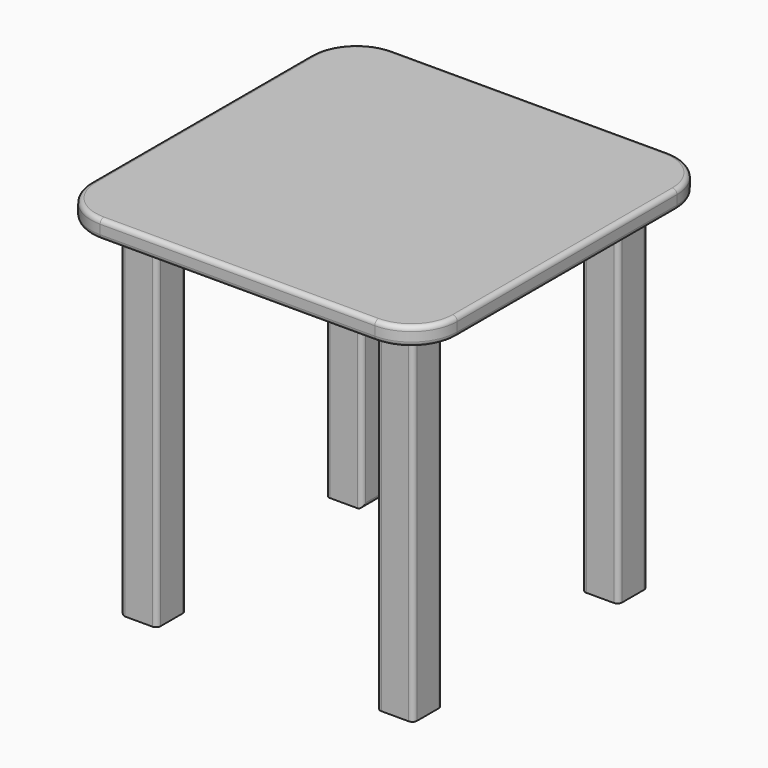
from build123d import *

# Parameters (mm, degrees)
F1_DEPTH = 20
F2_R     = 5
F3_W     = 40
F3_H     = 40
F4_DEPTH = 380
F5_F1_R  = 5
F5_F2_R  = 5
F6_R     = 5


with BuildPart() as f1:
    # F0 (on Top) → F1 (new body)
    with BuildSketch(Plane.XY):
        with BuildLine():
            Line((105.9260419756, 203.463898824), (-194.0739580244, 203.463898824))
            ThreePointArc((-194.0739580244, 203.463898824), (-229.4292970837, 188.8192378834), (-244.0739580244, 153.463898824))
            Line((-244.0739580244, 153.463898824), (-244.0739580244, -146.536101176))
            ThreePointArc((-244.0739580244, -146.536101176), (-229.4292970837, -181.8914402353), (-194.0739580244, -196.536101176))
            Line((-194.0739580244, -196.536101176), (105.9260419756, -196.536101176))
            ThreePointArc((105.9260419756, -196.536101176), (141.2813810349, -181.8914402353), (155.9260419756, -146.536101176))
            Line((155.9260419756, -146.536101176), (155.9260419756, 153.463898824))
            ThreePointArc((155.9260419756, 153.463898824), (141.2813810349, 188.8192378834), (105.9260419756, 203.463898824))
        make_face()
    extrude(amount=F1_DEPTH)

    # F2
    f2_edges = [f1.edges().sort_by_distance(p)[0] for p in [
        (-44.073958, 203.463899, 0),
        (-229.429297, 188.819238, 0),
        (-244.073958, 3.463899, 0),
        (-229.429297, -181.89144, 0),
        (-44.073958, -196.536101, 0),
        (141.281381, -181.89144, 0),
        (155.926042, 3.463899, 0),
        (141.281381, 188.819238, 0),
    ]]
    fillet(f2_edges, radius=F2_R)

    # F3 (on face) → F4 (join)
    with BuildSketch(Plane(origin=(0, 0, 0), x_dir=(1, 0, 0), z_dir=(0, 0, -1))):
        with Locations((95.9260419756, 136.536101176)):
            Rectangle(F3_W, F3_H)
        with Locations((95.9260419756, -143.463898824)):
            Rectangle(F3_W, F3_H)
        with Locations((-184.0739580244, -143.463898824)):
            Rectangle(F3_W, F3_H)
        with Locations((-184.0739580244, 136.536101176)):
            Rectangle(F3_W, F3_H)
    extrude(amount=F4_DEPTH)

    # F5: fillet of radius 5 on 20 edges, made by hand

    # F5_f1
    f5_f1_edges = [f1.edges().sort_by_distance(p)[0] for p in [
        (-164.0739580244, -156.536101176, -190),
        (-164.0739580244, -116.536101176, -190),
        (-204.0739580244, -156.536101176, -190),
        (-204.0739580244, -116.536101176, -190),
        (-204.0739580244, -136.536101176, -380),
        (75.9260419756, -156.536101176, -190),
        (115.9260419756, -156.536101176, -190),
        (115.9260419756, -116.536101176, -190),
        (75.9260419756, -116.536101176, -190),
        (115.9260419756, 123.463898824, -190),
        (115.9260419756, 163.463898824, -190),
        (75.9260419756, 163.463898824, -190),
        (75.9260419756, 123.463898824, -190),
        (-204.0739580244, 163.463898824, -190),
        (-204.0739580244, 123.463898824, -190),
        (-164.0739580244, 163.463898824, -190),
        (-164.0739580244, 123.463898824, -190),
        (-164.0739580244, 143.463898824, -380),
    ]]
    fillet(f5_f1_edges, radius=F5_F1_R)

    # F5_f2
    f5_f2_edges = [f1.edges().sort_by_distance(p)[0] for p in [
        (-204.0739580244, -136.536101176, 0),
        (-164.0739580244, 143.463898824, 0),
        (-165.5384241184, 161.99943273, 0),
        (-165.5384241184, 124.9283649181, 0),
        (-202.6094919303, -155.0716350819, 0),
        (-202.6094919303, -118.00056727, 0),
    ]]
    fillet(f5_f2_edges, radius=F5_F2_R)

    # F6
    f6_edges = [f1.edges().sort_by_distance(p)[0] for p in [
        (-44.073958, 203.463899, 20),
        (-229.429297, 188.819238, 20),
        (-244.073958, 3.463899, 20),
        (-229.429297, -181.89144, 20),
        (-44.073958, -196.536101, 20),
        (141.281381, -181.89144, 20),
        (155.926042, 3.463899, 20),
        (141.281381, 188.819238, 20),
    ]]
    fillet(f6_edges, radius=F6_R)


solid = f1.part
